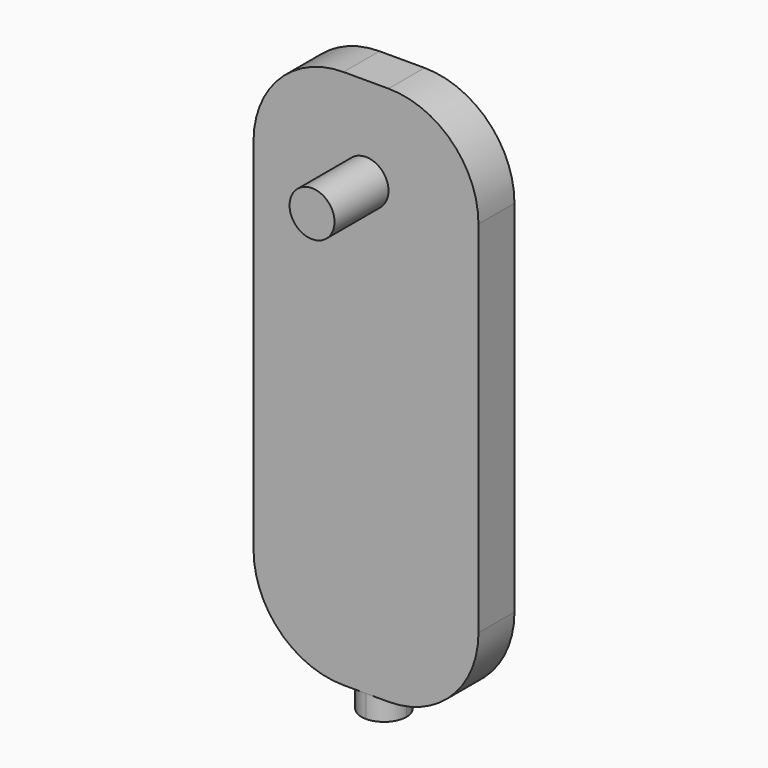
from build123d import *

# Parameters (mm, degrees)
F0_W     = 50
F0_H     = 10
F1_DEPTH = 120
F2_R     = 5
F3_DEPTH = 15
F5_DEPTH = 5
F6_R     = 19.99999


# Not quite as in the source:
# - a fillet or chamfer is up to 0.001 mm smaller than in the source, because OpenCascade refuses the exact size


with BuildPart() as f1:
    # F0 (on Top) → F1 (new body)
    with BuildSketch(Plane.XY):
        Rectangle(F0_W, F0_H)
    extrude(amount=F1_DEPTH)

    # F2 (on face) → F3 (join)
    with BuildSketch(Plane.XZ.offset(5)):
        with Locations((0, 100)):
            Circle(F2_R)
    extrude(amount=F3_DEPTH)

    # F4 (on face) → F5 (join)
    with BuildSketch(Plane(origin=(0, 0, 0), x_dir=(1, 0, 0), z_dir=(0, 0, -1))):
        with BuildLine():
            ThreePointArc((-3.84e-08, -5), (3.5355338924, -3.5355339195), (5, 0))
            ThreePointArc((5, 0), (3.5355339085, 3.5355339034), (7.2e-09, 5))
            ThreePointArc((7.2e-09, 5), (-5, 2.28e-08), (-3.84e-08, -5))
        make_face()
    extrude(amount=F5_DEPTH)

    # F6 (radius 20 in the source; OpenCascade refuses exactly that, so slightly less here)
    f6_edges = [f1.edges().sort_by_distance(p)[0] for p in [
        (25, 0, 0),
        (-25, 0, 0),
        (-25, 0, 120),
        (25, 0, 120),
    ]]
    fillet(f6_edges, radius=F6_R)


solid = f1.part
